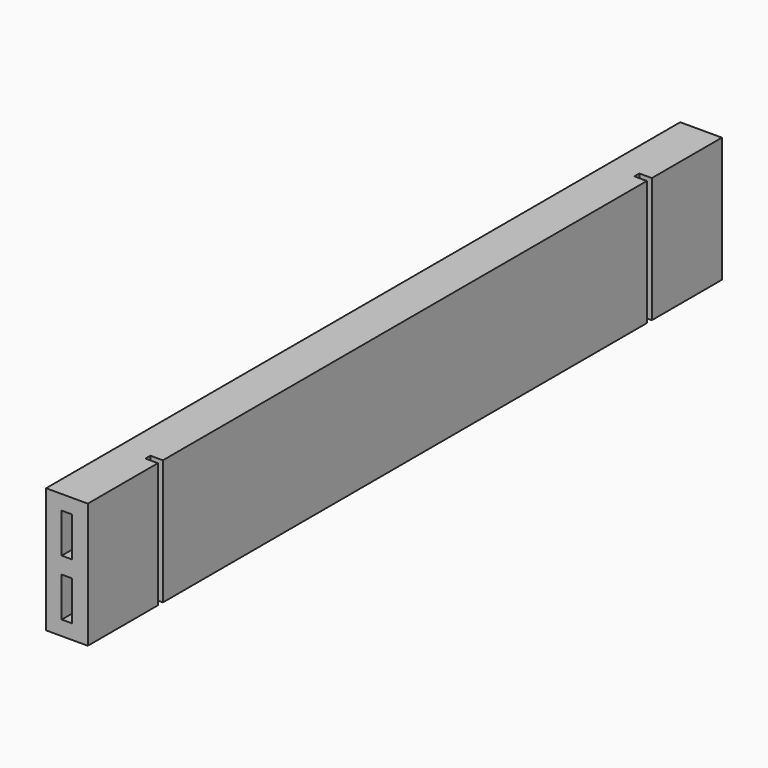
from build123d import *

# Parameters (mm, degrees)
F1_DEPTH = 20
F2_W     = 6
F2_H     = 3
F3_DEPTH = 60
F4_W     = 5
F4_H     = 19
F5_DEPTH = 15
F6_W     = 5
F6_H     = 19
F7_DEPTH = 15


# Not quite as in the source:
# - a feature names something its author has since deleted; it is built from what else it names


with BuildPart() as f1:
    # F0 (on Right) → F1 (new body)
    with BuildSketch(Plane.YZ):
        Polygon((190, 0), (-190, 0), (-190, -60), (0, -60), (190, -60), align=None)
    extrude(amount=F1_DEPTH)

    # F2 (on face) → F3 (cut)
    with BuildSketch(Plane(origin=(0, 0, -60), x_dir=(1, 0, 0), z_dir=(0, 0, -1))):
        with Locations((17, 146.5)):
            Rectangle(F2_W, F2_H)
        with Locations((17, -146.5)):
            Rectangle(F2_W, F2_H)
    extrude(amount=-F3_DEPTH, mode=Mode.SUBTRACT)

    # F4 (on face) → F5 (cut)
    with BuildSketch(Plane.XZ.offset(190)):
        with Locations((10, -16.5)):
            Rectangle(F4_W, F4_H)
        with Locations((10, -43.5)):
            Rectangle(F4_W, F4_H)
    extrude(amount=-F5_DEPTH, mode=Mode.SUBTRACT)

    # F6 (on face) → F7 (cut)
    with BuildSketch(Plane(origin=(0, 190, 0), x_dir=(-1, 0, 0), z_dir=(0, 1, 0))):
        with Locations((-10, -16.5)):
            Rectangle(F6_W, F6_H)
        with Locations((-10, -43.5)):
            Rectangle(F6_W, F6_H)
    extrude(amount=-F7_DEPTH, mode=Mode.SUBTRACT)


solid = f1.part
